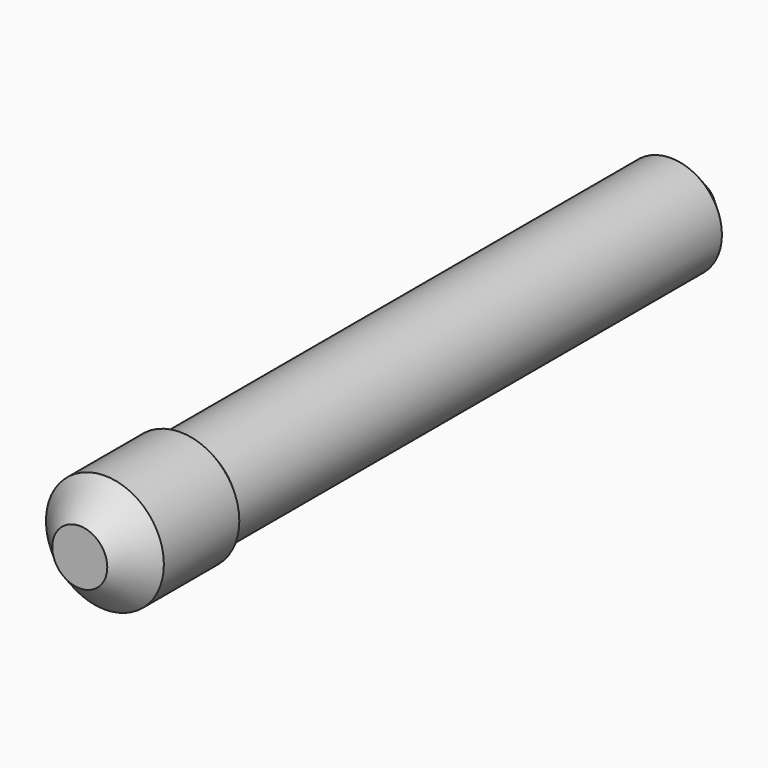
from build123d import *

# Parameters (mm, degrees)
F0_R        = 8.255
F1_DEPTH    = 99.06
F2_R        = 9.525
F3_DEPTH    = 25.4
F4_S5_R     = 8.255
F4_T6_DEPTH = 15
F5_SIZE     = 5.08


# Not quite as in the source:
# - a fillet or chamfer that OpenCascade refuses, or shapes differently, is made with other operations: its cross-section is extruded or revolved along the edge and cut away or added


with BuildPart() as f1:
    # F0 (on Front) → F1 (new body)
    with BuildSketch(Plane.XZ):
        Circle(F0_R)
    extrude(amount=F1_DEPTH)

    # F2 (on face) → F3 (join)
    with BuildSketch(Plane.XZ.offset(99.06)):
        Circle(F2_R)
    extrude(amount=F3_DEPTH)

    # F4: chamfer of 5.08 on 3 edges, made by hand


with BuildPart() as f4_tool2:
    # F4_s3 → F4_t4 (revolve)
    with BuildSketch(Plane.XY):
        Polygon((9.525, -104.14), (4.445, -99.06), (9.525, -99.06), align=None)
    revolve(axis=Axis((0, -99.06, 0), (0, -1, 0)))

    # F4_s5 → F4_t6 (cut, symmetric)
    with BuildSketch(Plane.XZ.offset(101.6)):
        Circle(F4_S5_R)
    extrude(amount=F4_T6_DEPTH, both=True, mode=Mode.SUBTRACT)


with BuildPart() as f1_1:
    add(f1.part)

    # F4_t1: cut F4_tool2
    add(f4_tool2.part, mode=Mode.SUBTRACT)

    # F4_s7 → F4_t8 (revolve, cut)
    with BuildSketch(Plane.XY):
        Polygon((9.525, -119.38), (4.445, -124.46), (9.525, -124.46), align=None)
    revolve(axis=Axis((0, -124.46, 0), (0, -1, 0)), mode=Mode.SUBTRACT)

    # F5
    f5_edges = [f1_1.edges().sort_by_distance(p)[0] for p in [
        (-8.255, 0, 0),
    ]]
    chamfer(f5_edges, length=F5_SIZE)


solid = f1_1.part
